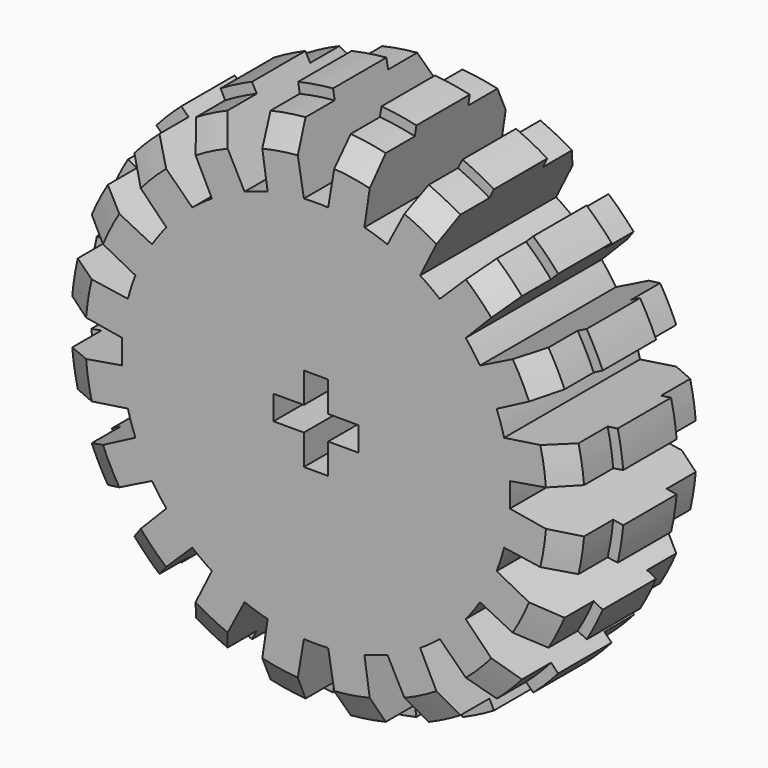
from build123d import *

# Parameters (mm, degrees)
F0_R            = 11
F1_DEPTH        = 7
F5_DEPTH        = 7.001
F5_COPIES_COUNT = 20


# Not quite as in the source:
# - a pattern or mirror of a feature is missing from the dataset's text; its kind, count and spacing are read off the source's solid


with BuildPart() as f1:
    # F0 (on Front) → F1 (new body)
    with BuildSketch(Plane.XZ):
        Circle(F0_R)
        Polygon((-1.75, 0.5), (-0.5, 0.5), (-0.5, 1.75), (0.5, 1.75), (0.5, 0.5), (1.75, 0.5), (1.75, -0.5), (0.5, -0.5), (0.5, -1.75), (-0.5, -1.75), (-0.5, -0.5), (-1.75, -0.5), align=None, mode=Mode.SUBTRACT)
    extrude(amount=F1_DEPTH)

    # F2 (on Right) → F3 (revolve, cut)
    with BuildSketch(Plane.YZ):
        Polygon((-7, 12.5), (-7, 9.5), (-6.375, 10.5825317547), (-4.875, 10.5825317547), (-4.875, 11), (-2.125, 11), (-2.125, 10.5825317547), (-0.625, 10.5825317547), (0, 9.5), (0, 12.5), align=None)
    revolve(axis=Axis((0, 2.603987056, 0), (0, 1, 0)), mode=Mode.SUBTRACT)

    # F4 (on Front) → F5 (cut, through all)
    with BuildSketch(Plane.XZ):
        with BuildLine():
            Line((0.5, 7.9843597113), (1, 10.9544511501))
            ThreePointArc((1, 10.9544511501), (0, 11), (-1, 10.9544511501))
            Line((-1, 10.9544511501), (-0.5, 7.9843597113))
            ThreePointArc((-0.5, 7.9843597113), (0, 8), (0.5, 7.9843597113))
        make_face()
    f5 = extrude(amount=F5_DEPTH, mode=Mode.SUBTRACT)

    # F5_copies: F5 ×20 about axis
    f5_copies_axis = Axis((0, 0, 0), (0, 1, 0))
    for i in range(1, F5_COPIES_COUNT):
        add(f5.rotate(f5_copies_axis, i * 360 / F5_COPIES_COUNT), mode=Mode.SUBTRACT)


solid = f1.part
